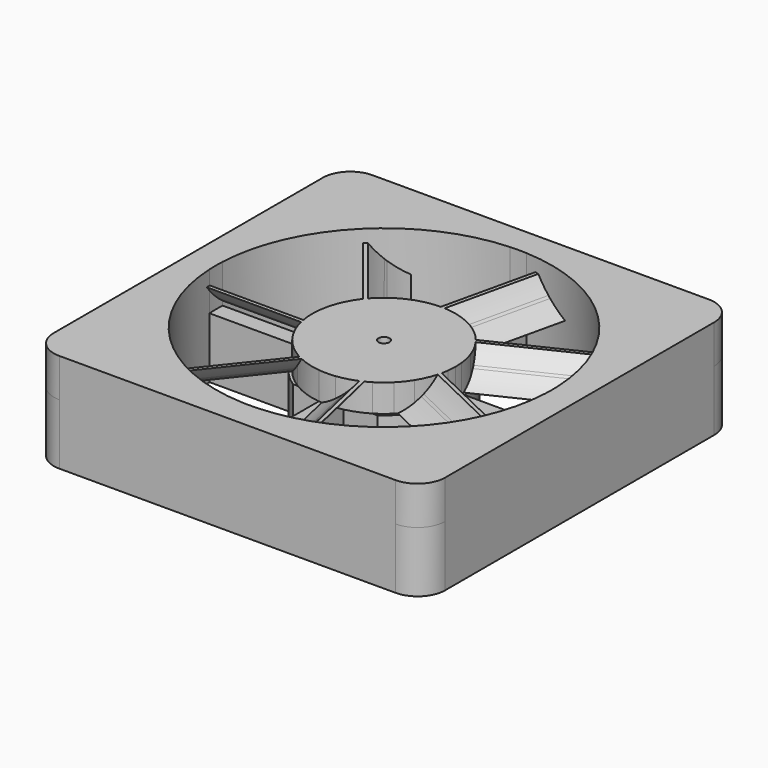
from build123d import *

# Parameters (mm, degrees)
F0_W      = 71
F0_H      = 71
F1_DEPTH  = 11
F2_R      = 5
F4_DEPTH  = 7
F6_DEPTH  = 5
F9_DEPTH  = 29.75
F10_COUNT = 7
F11_R     = 1
F12_DEPTH = 7.2


with BuildPart() as f1:
    # F0 (on Top) → F1 (new body)
    with BuildSketch(Plane.XY):
        with Locations((6.5, -7.6)):
            Rectangle(F0_W, F0_H)
        with BuildLine():
            ThreePointArc((36.9630924235, -6.1), (36.9907717098, -6.8497730061), (37, -7.6))
            ThreePointArc((37, -7.6), (36.9907717098, -8.3502269939), (36.9630924235, -9.1))
            ThreePointArc((36.9630924235, -9.1), (28.0667568262, -29.1667568262), (8, -38.0630924235))
            ThreePointArc((8, -38.0630924235), (6.5, -38.1), (5, -38.0630924235))
            ThreePointArc((5, -38.0630924235), (-15.0667568262, -29.1667568262), (-23.9630924235, -9.1))
            ThreePointArc((-23.9630924235, -9.1), (-24, -7.6), (-23.9630924235, -6.1))
            ThreePointArc((-23.9630924235, -6.1), (-15.0667568262, 13.9667568262), (5, 22.8630924235))
            ThreePointArc((5, 22.8630924235), (6.5, 22.9), (8, 22.8630924235))
            ThreePointArc((8, 22.8630924235), (28.0667568262, 13.9667568262), (36.9630924235, -6.1))
        make_face(mode=Mode.SUBTRACT)
        with BuildLine():
            Line((-7.05, -6.1), (-23.9630924235, -6.1))
            ThreePointArc((-23.9630924235, -6.1), (-24, -7.6), (-23.9630924235, -9.1))
            Line((-23.9630924235, -9.1), (-7.05, -9.1))
            Line((-7.05, -9.1), (-6.9658446471, -9.1))
            ThreePointArc((-6.9658446471, -9.1), (-7.05, -7.6), (-6.9658446471, -6.1))
            Line((-6.9658446471, -6.1), (-7.05, -6.1))
        make_face()
        with BuildLine():
            Line((14.1646652259, 3.5), (8, 3.5))
            Line((8, 3.5), (5, 3.5))
            Line((5, 3.5), (-1.1646652259, 3.5))
            ThreePointArc((-1.1646652259, 3.5), (-5.1171728234, -0.6643370418), (-6.9658446471, -6.1))
            ThreePointArc((-6.9658446471, -6.1), (-7.05, -7.6), (-6.9658446471, -9.1))
            ThreePointArc((-6.9658446471, -9.1), (-5.1171728234, -14.5356629582), (-1.1646652259, -18.7))
            Line((-1.1646652259, -18.7), (5, -18.7))
            Line((5, -18.7), (8, -18.7))
            Line((8, -18.7), (14.1646652259, -18.7))
            ThreePointArc((14.1646652259, -18.7), (18.1171728234, -14.5356629582), (19.9658446471, -9.1))
            ThreePointArc((19.9658446471, -9.1), (20.05, -7.6), (19.9658446471, -6.1))
            ThreePointArc((19.9658446471, -6.1), (18.1171728234, -0.6643370418), (14.1646652259, 3.5))
        make_face()
        with BuildLine():
            ThreePointArc((0, -15.2), (-3.55, -7.6), (0, 0))
            Line((0, 0), (6.5, 0))
            Line((6.5, 0), (13, 0))
            ThreePointArc((13, 0), (16.55, -7.6), (13, -15.2))
            Line((13, -15.2), (6.5, -15.2))
            Line((6.5, -15.2), (0, -15.2))
        make_face(mode=Mode.SUBTRACT)
        with BuildLine():
            Line((8, 3.5), (8, 22.8630924235))
            ThreePointArc((8, 22.8630924235), (6.5, 22.9), (5, 22.8630924235))
            Line((5, 22.8630924235), (5, 3.5))
            Line((5, 3.5), (8, 3.5))
        make_face()
        with BuildLine():
            ThreePointArc((36.9630924235, -9.1), (36.9907717098, -8.3502269939), (37, -7.6))
            ThreePointArc((37, -7.6), (36.9907717098, -6.8497730061), (36.9630924235, -6.1))
            Line((36.9630924235, -6.1), (20.05, -6.1))
            Line((20.05, -6.1), (19.9658446471, -6.1))
            ThreePointArc((19.9658446471, -6.1), (20.05, -7.6), (19.9658446471, -9.1))
            Line((19.9658446471, -9.1), (20.05, -9.1))
            Line((20.05, -9.1), (36.9630924235, -9.1))
        make_face()
        with BuildLine():
            ThreePointArc((5, -38.0630924235), (6.5, -38.1), (8, -38.0630924235))
            Line((8, -38.0630924235), (8, -18.7))
            Line((8, -18.7), (5, -18.7))
            Line((5, -18.7), (5, -38.0630924235))
        make_face()
    extrude(amount=F1_DEPTH)

    # F2
    f2_edges = [f1.edges().sort_by_distance(p)[0] for p in [
        (-29, 27.9, 5.5),
        (42, 27.9, 5.5),
        (42, -43.1, 5.5),
        (-29, -43.1, 5.5),
    ]]
    fillet(f2_edges, radius=F2_R)

    # F3 (on face) → F4 (join)
    with BuildSketch(Plane.XY.offset(11)):
        with BuildLine():
            Line((37, 27.9), (-24, 27.9))
            ThreePointArc((-24, 27.9), (-27.5355339059, 26.4355339059), (-29, 22.9))
            Line((-29, 22.9), (-29, -38.1))
            ThreePointArc((-29, -38.1), (-27.5355339059, -41.6355339059), (-24, -43.1))
            Line((-24, -43.1), (37, -43.1))
            ThreePointArc((37, -43.1), (40.5355339059, -41.6355339059), (42, -38.1))
            Line((42, -38.1), (42, 22.9))
            ThreePointArc((42, 22.9), (40.5355339059, 26.4355339059), (37, 27.9))
        make_face()
        with BuildLine():
            ThreePointArc((36.9630924235, -6.1), (36.9907717098, -6.8497730061), (37, -7.6))
            ThreePointArc((37, -7.6), (36.9907717098, -8.3502269939), (36.9630924235, -9.1))
            ThreePointArc((36.9630924235, -9.1), (28.0667568262, -29.1667568262), (8, -38.0630924235))
            ThreePointArc((8, -38.0630924235), (6.5, -38.1), (5, -38.0630924235))
            ThreePointArc((5, -38.0630924235), (-15.0667568262, -29.1667568262), (-23.9630924235, -9.1))
            ThreePointArc((-23.9630924235, -9.1), (-24, -7.6), (-23.9630924235, -6.1))
            ThreePointArc((-23.9630924235, -6.1), (-15.0667568262, 13.9667568262), (5, 22.8630924235))
            ThreePointArc((5, 22.8630924235), (6.5, 22.9), (8, 22.8630924235))
            ThreePointArc((8, 22.8630924235), (28.0667568262, 13.9667568262), (36.9630924235, -6.1))
        make_face(mode=Mode.SUBTRACT)
    extrude(amount=F4_DEPTH)


with BuildPart() as f6:
    # F5 (on face) → F6 (new body)
    with BuildSketch(Plane.XY.offset(11)):
        with BuildLine():
            ThreePointArc((13.2668308683, -18.7), (17.8350959698, -13.9651865139), (19.5, -7.6))
            ThreePointArc((19.5, -7.6), (17.8350959698, -1.2348134861), (13.2668308683, 3.5))
            Line((13.2668308683, 3.5), (8, 3.5))
            Line((8, 3.5), (8, 5.3131715701))
            ThreePointArc((8, 5.3131715701), (6.5, 5.4), (5, 5.3131715701))
            Line((5, 5.3131715701), (5, 3.5))
            Line((5, 3.5), (-0.2668308683, 3.5))
            ThreePointArc((-0.2668308683, 3.5), (-6.5, -7.6), (-0.2668308683, -18.7))
            Line((-0.2668308683, -18.7), (5, -18.7))
            Line((5, -18.7), (5, -20.5131715701))
            ThreePointArc((5, -20.5131715701), (6.5, -20.6), (8, -20.5131715701))
            Line((8, -20.5131715701), (8, -18.7))
            Line((8, -18.7), (13.2668308683, -18.7))
        make_face()
        with BuildLine():
            Line((0, 0), (13, 0))
            ThreePointArc((13, 0), (16.55, -7.6), (13, -15.2))
            Line((13, -15.2), (0, -15.2))
            ThreePointArc((0, -15.2), (-3.55, -7.6), (0, 0))
        make_face(mode=Mode.SUBTRACT)
        with BuildLine():
            ThreePointArc((13, -15.2), (16.55, -7.6), (13, 0))
            Line((13, 0), (0, 0))
            ThreePointArc((0, 0), (-3.55, -7.6), (0, -15.2))
            Line((0, -15.2), (13, -15.2))
        make_face()
        with BuildLine():
            Line((5, 3.5), (5, 5.3131715701))
            ThreePointArc((5, 5.3131715701), (2.2683311877, 4.6919884097), (-0.2668308683, 3.5))
            Line((-0.2668308683, 3.5), (5, 3.5))
        make_face()
        with BuildLine():
            Line((8, 3.5), (13.2668308683, 3.5))
            ThreePointArc((13.2668308683, 3.5), (10.7316688123, 4.6919884097), (8, 5.3131715701))
            Line((8, 5.3131715701), (8, 3.5))
        make_face()
        with BuildLine():
            ThreePointArc((-0.2668308683, -18.7), (2.2683311877, -19.8919884097), (5, -20.5131715701))
            Line((5, -20.5131715701), (5, -18.7))
            Line((5, -18.7), (-0.2668308683, -18.7))
        make_face()
        with BuildLine():
            ThreePointArc((8, -20.5131715701), (10.7316688123, -19.8919884097), (13.2668308683, -18.7))
            Line((13.2668308683, -18.7), (8, -18.7))
            Line((8, -18.7), (8, -20.5131715701))
        make_face()
    extrude(amount=F6_DEPTH)

    # F8 (on offset) → F9 (join)
    with BuildSketch(Plane.YZ.offset(6.5)):
        with BuildLine():
            ThreePointArc((-7.990379433, 13.174815303), (-7.7964841083, 13.0139604512), (-7.6, 12.8562782535))
            Line((-7.6, 12.8562782535), (-7.6, 13.5080789351))
            ThreePointArc((-7.6, 13.5080789351), (-7.7939088019, 13.3399466771), (-7.990379433, 13.174815303))
        make_face()
        with BuildLine():
            Line((-7.6, 13.5080789351), (-7.6, 12.8562782535))
            ThreePointArc((-7.6, 12.8562782535), (-7.4035158917, 13.0139604512), (-7.209620567, 13.174815303))
            ThreePointArc((-7.209620567, 13.174815303), (-7.4060911981, 13.3399466771), (-7.6, 13.5080789351))
        make_face()
        with BuildLine():
            ThreePointArc((-7.209620567, 13.174815303), (-7.4035158917, 13.0139604512), (-7.6, 12.8562782535))
            ThreePointArc((-7.6, 12.8562782535), (-6.152984063, 11.8425096212), (-4.6, 11))
            Line((-4.6, 11), (-3.8189750324, 11))
            ThreePointArc((-3.8189750324, 11), (-5.5801347672, 11.9847645353), (-7.209620567, 13.174815303))
        make_face()
        with BuildLine():
            ThreePointArc((-7.990379433, 13.174815303), (-7.7939088019, 13.3399466771), (-7.6, 13.5080789351))
            ThreePointArc((-7.6, 13.5080789351), (-8.8170720896, 14.6952230489), (-9.9070871014, 16))
            Line((-9.9070871014, 16), (-10.6, 16))
            ThreePointArc((-10.6, 16), (-9.3831560319, 14.506153245), (-7.990379433, 13.174815303))
        make_face()
    extrude(amount=-F9_DEPTH)

    # F10: F6 ×7 about axis
    f10_axis = Axis((6.5, -7.6, 13.5), (0, 0, 1))


with BuildPart() as f6_1:
    add(f6.part)
    for i in range(1, F10_COUNT):
        add(f6.part.rotate(f10_axis, i * 360 / F10_COUNT))

    # F11 (on face) → F12 (cut)
    with BuildSketch(Plane.XY.offset(11)):
        with Locations((6.5, -7.6)):
            Circle(F11_R)
    extrude(amount=F12_DEPTH, mode=Mode.SUBTRACT)


solid = Compound([f1.part, f6_1.part])
